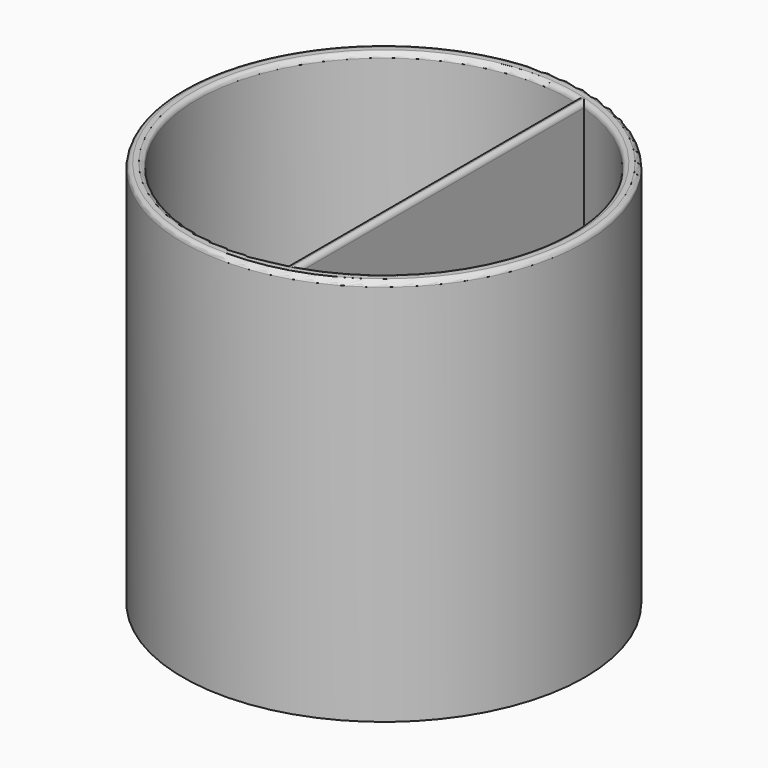
from build123d import *

# Parameters (mm, degrees)
F0_R     = 38.5
F2_DEPTH = 5
F0_R_2   = 41.5
F1_W     = 2
F1_H     = 74.3572457801
F3_DEPTH = 80
F5_DEPTH = 3
F6_R     = 0.99999


# Not quite as in the source:
# - a fillet or chamfer is up to 0.001 mm smaller than in the source, because OpenCascade refuses the exact size


with BuildPart() as f2:
    # F0 (on Top) → F2 (new body)
    with BuildSketch(Plane.XY):
        Circle(F0_R)
    extrude(amount=F2_DEPTH)

    # F0 (on Top) + F1 (on Top) → F3 (join)
    with BuildSketch(Plane.XY):
        Circle(F0_R_2)
        Circle(F0_R, mode=Mode.SUBTRACT)
    with BuildSketch(Plane.XY):
        with Locations((11, 0)):
            Rectangle(F1_W, F1_H)
    extrude(amount=F3_DEPTH)

    # F4 (on Top) → F5 (cut)
    with BuildSketch(Plane.XY):
        Polygon((0, -3), (-4, -38), (4, -38), align=None)
        Polygon((15.5468718514, -34.9040796417), (0.9270509831, -2.8531695489), (7.9384197211, -37.3762155967), align=None)
        Polygon((25.5719075646, -28.3915047771), (1.7633557569, -2.4270509831), (19.0997716096, -33.0937867954), align=None)
        Polygon((33.0937867954, -19.0997716096), (2.4270509831, -1.7633557569), (28.3915047771, -25.5719075646), align=None)
        Polygon((37.3762155967, -7.9384197211), (2.8531695489, -0.9270509831), (34.9040796417, -15.5468718514), align=None)
        Polygon((38, 4), (3, 0), (38, -4), align=None)
        Polygon((34.9040796417, 15.5468718514), (2.8531695489, 0.9270509831), (37.3762155967, 7.9384197211), align=None)
        Polygon((28.3915047771, 25.5719075646), (2.4270509831, 1.7633557569), (33.0937867954, 19.0997716096), align=None)
        Polygon((19.0997716096, 33.0937867954), (1.7633557569, 2.4270509831), (25.5719075646, 28.3915047771), align=None)
        Polygon((7.9384197211, 37.3762155967), (0.9270509831, 2.8531695489), (15.5468718514, 34.9040796417), align=None)
        Polygon((-4, 38), (0, 3), (4, 38), align=None)
        Polygon((-15.5468718514, 34.9040796417), (-0.9270509831, 2.8531695489), (-7.9384197211, 37.3762155967), align=None)
        Polygon((-25.5719075646, 28.3915047771), (-1.7633557569, 2.4270509831), (-19.0997716096, 33.0937867954), align=None)
        Polygon((-33.0937867954, 19.0997716096), (-2.4270509831, 1.7633557569), (-28.3915047771, 25.5719075646), align=None)
        Polygon((-37.3762155967, 7.9384197211), (-2.8531695489, 0.9270509831), (-34.9040796417, 15.5468718514), align=None)
        Polygon((-38, -4), (-3, 0), (-38, 4), align=None)
        Polygon((-34.9040796417, -15.5468718514), (-2.8531695489, -0.9270509831), (-37.3762155967, -7.9384197211), align=None)
        Polygon((-28.3915047771, -25.5719075646), (-2.4270509831, -1.7633557569), (-33.0937867954, -19.0997716096), align=None)
        Polygon((-19.0997716096, -33.0937867954), (-1.7633557569, -2.4270509831), (-25.5719075646, -28.3915047771), align=None)
        Polygon((-7.9384197211, -37.3762155967), (-0.9270509831, -2.8531695489), (-15.5468718514, -34.9040796417), align=None)
    extrude(amount=F5_DEPTH, mode=Mode.SUBTRACT)

    # F6 (radius 1 in the source; OpenCascade refuses exactly that, so slightly less here)
    f6_edges = [f2.edges().sort_by_distance(p)[0] for p in [
        (-38.5, 0, 80),
        (-41.5, 0, 80),
        (12, 0, 80),
        (10, 0, 80),
        (38.5, 0, 80),
    ]]
    fillet(f6_edges, radius=F6_R)


solid = f2.part
